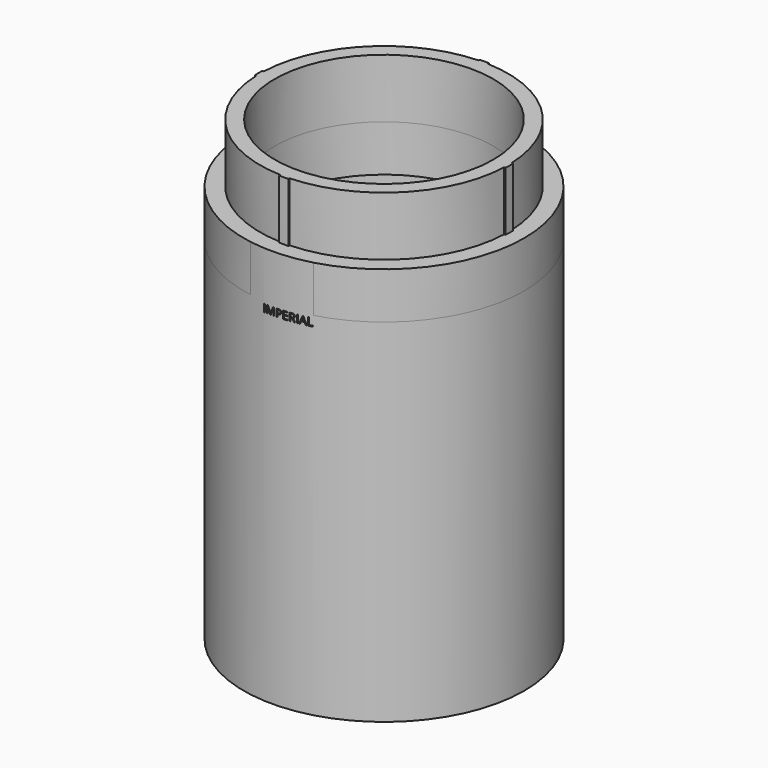
from build123d import *

# Parameters (mm, degrees)
F0_R         = 11.75385
F1_DEPTH     = 6.35
F2_R         = 15.08125
F2_R_2       = 13.49375
F3_DEPTH     = 42.8625
F4_R         = 15.08125
F4_R_2       = 11.75385
F5_DEPTH     = 5
F6_TEXT_SIZE = 1.1453523748
F7_DEPTH     = 127


# Not quite as in the source:
# - Text() gives the source's letters only with a copy of the font that has no kerning and outlines rounded to 1/6400 em; it was checked with that copy


with BuildPart() as f1:
    # F0 (on Top) → F1 (new body)
    with BuildSketch(Plane.XY):
        with BuildLine():
            ThreePointArc((13.3319773411, -0.5), (13.3390066295, -0.2500439195), (13.34135, 0))
            ThreePointArc((13.34135, 0), (13.3390066295, 0.2500439195), (13.3319773411, 0.5))
            ThreePointArc((13.3319773411, 0.5), (9.4337590552, 9.4337590552), (0.5, 13.3319773411))
            ThreePointArc((0.5, 13.3319773411), (0, 13.34135), (-0.5, 13.3319773411))
            ThreePointArc((-0.5, 13.3319773411), (-9.4337590552, 9.4337590552), (-13.3319773411, 0.5))
            ThreePointArc((-13.3319773411, 0.5), (-13.34135, 0), (-13.3319773411, -0.5))
            ThreePointArc((-13.3319773411, -0.5), (-9.4337590552, -9.4337590552), (-0.5, -13.3319773411))
            ThreePointArc((-0.5, -13.3319773411), (0, -13.34135), (0.5, -13.3319773411))
            ThreePointArc((0.5, -13.3319773411), (9.4337590552, -9.4337590552), (13.3319773411, -0.5))
        make_face()
        Circle(F0_R, mode=Mode.SUBTRACT)
        with BuildLine():
            ThreePointArc((13.3319773411, 0.5), (13.3390066295, 0.2500439195), (13.34135, 0))
            ThreePointArc((13.34135, 0), (13.3390066295, -0.2500439195), (13.3319773411, -0.5))
            Line((13.3319773411, -0.5), (13.4844832701, -0.5))
            ThreePointArc((13.4844832701, -0.5), (13.49375, 0), (13.4844832701, 0.5))
            Line((13.4844832701, 0.5), (13.3319773411, 0.5))
        make_face()
        with BuildLine():
            ThreePointArc((-0.5, 13.3319773411), (0, 13.34135), (0.5, 13.3319773411))
            Line((0.5, 13.3319773411), (0.5, 13.4844832701))
            ThreePointArc((0.5, 13.4844832701), (0, 13.49375), (-0.5, 13.4844832701))
            Line((-0.5, 13.4844832701), (-0.5, 13.3319773411))
        make_face()
        with BuildLine():
            Line((0.5, -13.4844832701), (0.5, -13.3319773411))
            ThreePointArc((0.5, -13.3319773411), (0, -13.34135), (-0.5, -13.3319773411))
            Line((-0.5, -13.3319773411), (-0.5, -13.4844832701))
            ThreePointArc((-0.5, -13.4844832701), (0, -13.49375), (0.5, -13.4844832701))
        make_face()
        with BuildLine():
            ThreePointArc((-13.3319773411, -0.5), (-13.34135, 0), (-13.3319773411, 0.5))
            Line((-13.3319773411, 0.5), (-13.4844832701, 0.5))
            ThreePointArc((-13.4844832701, 0.5), (-13.49375, 0), (-13.4844832701, -0.5))
            Line((-13.4844832701, -0.5), (-13.3319773411, -0.5))
        make_face()
    extrude(amount=F1_DEPTH)

    # F2 (on Top) → F3 (join)
    with BuildSketch(Plane.XY):
        Circle(F2_R)
        Circle(F2_R_2, mode=Mode.SUBTRACT)
    extrude(amount=-F3_DEPTH)

    # F6 (on Front) → F7 (cut)
    with BuildSketch(Plane.XZ):
        with Locations((-0.9830530764, -6.0762903381)):
            Text('IMPERIAL', F6_TEXT_SIZE, font='Open Sans', text_align=(TextAlign.LEFT, TextAlign.BOTTOM))
    extrude(amount=F7_DEPTH, mode=Mode.SUBTRACT)


with BuildPart() as f5:
    # F4 (on Top) → F5 (new body)
    with BuildSketch(Plane.XY):
        Circle(F4_R)
        Circle(F4_R_2, mode=Mode.SUBTRACT)
    extrude(amount=-F5_DEPTH)


solid = Compound([f1.part, f5.part])
